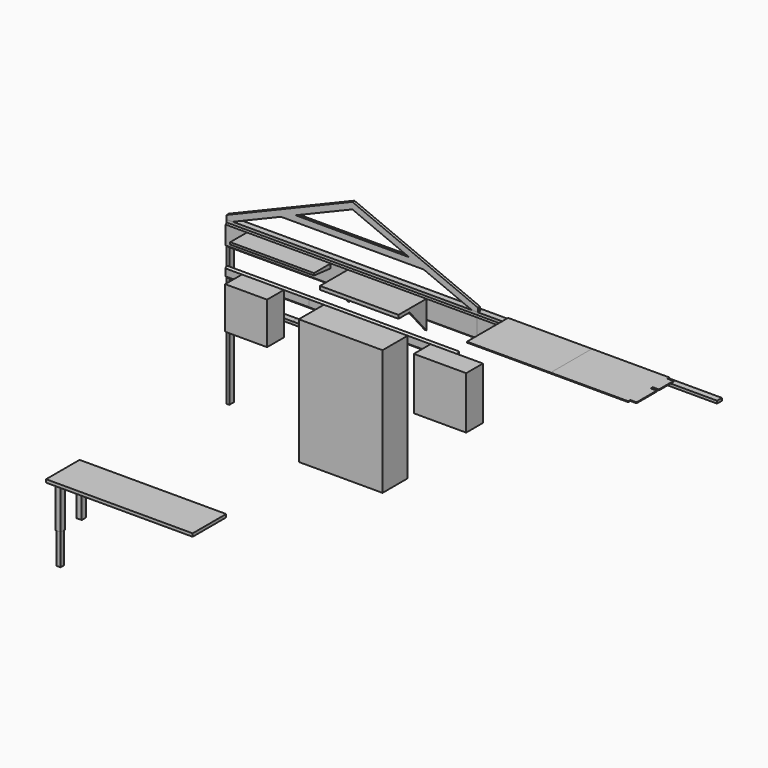
from build123d import *

# Parameters (mm, degrees)
F0_W      = 38.1
F0_H      = 88.9
F1_DEPTH  = 2324.1
F2_W      = 88.9
F2_H      = 38.1
F3_DEPTH  = 3657.6
F5_DEPTH  = 2438.4
F6_DEPTH  = 1219.2
F8_DEPTH  = 1219.2
F9_W      = 88.9
F9_H      = 38.1
F10_DEPTH = 914.4
F11_DEPTH = 1028.7
F12_DEPTH = 1028.7
F13_W     = 609.6
F13_H     = 609.6
F14_DEPTH = 304.8
F15_W     = 1219.2
F15_H     = 1828.8
F16_DEPTH = 457.2
F17_W     = 762
F17_H     = 762
F18_DEPTH = 304.8
F19_W     = 1219.2
F19_H     = 63.5
F20_DEPTH = 304.8
F22_DEPTH = 1529.2895152817
F23_W     = 1143
F23_H     = 50.8
F24_DEPTH = 508
F26_DEPTH = 25.4
F28_DEPTH = 25.4
F29_DEPTH = 1130.3
F30_W     = 1219.2
F30_H     = 749.3
F31_DEPTH = 12.7
F32_DEPTH = 3479.8
F33_DEPTH = 1130.3
F34_DEPTH = 635
F35_W     = 266.7
F35_H     = 12.7
F35_W_2   = 368.3
F36_DEPTH = 88.9
F37_W     = 2133.6
F37_H     = 609.6
F38_DEPTH = 44.45
F40_DEPTH = 38.1
F42_DEPTH = 6.35
F43_W     = 76.2
F43_H     = 76.2
F44_DEPTH = 609.6
F45_T     = -6.35
F46_W     = 58.42
F46_H     = 58.42
F47_DEPTH = 457.2
F48_T     = -2.54


with BuildPart() as f1:
    # F0 (on Top) → F1 (new body)
    with BuildSketch(Plane.XY):
        with Locations((19.05, -44.45)):
            Rectangle(F0_W, F0_H)
    extrude(amount=F1_DEPTH)


with BuildPart() as f3:
    # F2 (on face) → F3 (new body)
    with BuildSketch(Plane(origin=(0, 0, 0), x_dir=(0, -1, 0), z_dir=(-1, 0, 0))):
        with Locations((44.45, 2343.15)):
            Rectangle(F2_W, F2_H)
    extrude(amount=-F3_DEPTH)


with BuildPart() as f5:
    # F4 (on face) → F5 (new body)
    with BuildSketch(Plane(origin=(0, 0, 0), x_dir=(0, -1, 0), z_dir=(-1, 0, 0))):
        Polygon((107.95, 2305.05), (88.9, 2324.1), (88.9, 2019.3), (107.95, 2038.35), align=None)
    extrude(amount=-F5_DEPTH)


with BuildPart() as f6:
    # F6 (new): a face of the model
    f6_faces = [f5.part.faces().sort_by_distance(p)[0] for p in [
        (2438.4, -98.2133333333, 2171.7),
    ]]
    extrude(f6_faces, amount=F6_DEPTH)


with BuildPart() as f8:
    # F7 (on face) → F8 (new body)
    with BuildSketch(Plane(origin=(0, 0, 0), x_dir=(0, -1, 0), z_dir=(-1, 0, 0))):
        Polygon((114.3, 1747.0956106186), (88.9, 1772.4956106186), (88.9, 1620.0956106186), (114.3, 1645.4956106186), align=None)
    extrude(amount=-F8_DEPTH)


with BuildPart() as f10:
    # F9 (on face) → F10 (new body)
    with BuildSketch(Plane.YZ.offset(38.1)):
        with Locations((-44.45, 1349.1220453262)):
            Rectangle(F9_W, F9_H)
    extrude(amount=F10_DEPTH)


with BuildPart() as f11:
    # F11 (new): a face of the model
    f11_faces = [f6.part.faces().sort_by_distance(p)[0] for p in [
        (3657.6, -98.2133333333, 2171.7),
    ]]
    extrude(f11_faces, amount=F11_DEPTH)


with BuildPart() as f12:
    # F12 (new): a face of the model
    f12_faces = [f8.part.faces().sort_by_distance(p)[0] for p in [
        (1219.2, -100.7533333333, 1696.2956106186),
    ]]
    extrude(f12_faces, amount=F12_DEPTH)


with BuildPart() as f14:
    # F13 (on face) → F14 (new body)
    with BuildSketch(Plane.XZ.offset(114.3)):
        with Locations((546.8414686203, 1442.2956106186)):
            Rectangle(F13_W, F13_H)
    extrude(amount=F14_DEPTH)


with BuildPart() as f16:
    # F15 (on face) → F16 (new body)
    with BuildSketch(Plane.XZ.offset(114.3)):
        with Locations((2044.3823858261, 832.6956106186)):
            Rectangle(F15_W, F15_H)
    extrude(amount=F16_DEPTH)


with BuildPart() as f18:
    # F17 (on face) → F18 (new body)
    with BuildSketch(Plane.XZ.offset(114.3)):
        with Locations((3368.7196163048, 1366.0956106186)):
            Rectangle(F17_W, F17_H)
    extrude(amount=F18_DEPTH)


with BuildPart() as f20:
    # F19 (on face) → F20 (new body)
    with BuildSketch(Plane.XZ.offset(107.95)):
        with Locations((919.6885152817, 2273.3)):
            Rectangle(F19_W, F19_H)
    extrude(amount=F20_DEPTH)

    # F21 (on face) → F22 (cut, through all)
    with BuildSketch(Plane.YZ.offset(1529.2885152817)):
        Polygon((-107.95, 2241.55), (-412.75, 2273.3), (-412.75, 2241.55), align=None)
    extrude(amount=-F22_DEPTH, mode=Mode.SUBTRACT)


with BuildPart() as f24:
    # F23 (on face) → F24 (new body)
    with BuildSketch(Plane.XZ.offset(107.95)):
        with Locations((2350.8992757797, 2279.65)):
            Rectangle(F23_W, F23_H)
    extrude(amount=F24_DEPTH)

    # F25 (on face) → F26 (join)
    with BuildSketch(Plane.YZ.offset(2922.3992757797)):
        Polygon((-107.95, 1898.65), (-107.95, 2254.25), (-412.75, 2254.25), align=None)
    extrude(amount=-F26_DEPTH)

    # F27 (on face) → F28 (join)
    with BuildSketch(Plane(origin=(1779.3992757797, 0, 0), x_dir=(0, -1, 0), z_dir=(-1, 0, 0))):
        Polygon((107.95, 2254.25), (107.95, 1898.65), (412.75, 2254.25), align=None)
    extrude(amount=-F28_DEPTH)


with BuildPart() as f29:
    # F29 (new): a face of the model
    f29_faces = [f12.part.faces().sort_by_distance(p)[0] for p in [
        (2247.9, -100.7533333333, 1696.2956106186),
    ]]
    extrude(f29_faces, amount=F29_DEPTH)


with BuildPart() as f31:
    # F30 (on face) → F31 (new body)
    with BuildSketch(Plane.XY.offset(2362.2)):
        with Locations((4634.7321610946, -374.65)):
            Rectangle(F30_W, F30_H)
    extrude(amount=F31_DEPTH)


with BuildPart() as f32:
    # F32 (new): a face of the model
    f32_faces = [f3.part.faces().sort_by_distance(p)[0] for p in [
        (3657.6, -44.45, 2343.15),
    ]]
    extrude(f32_faces, amount=F32_DEPTH)


with BuildPart() as f33:
    # F33 (new): a face of the model
    f33_faces = [f31.part.faces().sort_by_distance(p)[0] for p in [
        (5244.3321610946, -374.65, 2368.55),
    ]]
    extrude(f33_faces, amount=F33_DEPTH)

    # F35 (on face) → F36 (join)
    with BuildSketch(Plane.YZ.offset(6374.6321610946)):
        with Locations((-171.45, 2368.55)):
            Rectangle(F35_W, F35_H)
        with Locations((-527.05, 2368.55)):
            Rectangle(F35_W_2, F35_H)
    extrude(amount=F36_DEPTH)


with BuildPart() as f34:
    # F34 (new): a face of the model
    f34_faces = [f10.part.faces().sort_by_distance(p)[0] for p in [
        (952.5, -44.45, 1349.1220453262),
    ]]
    extrude(f34_faces, amount=F34_DEPTH)


with BuildPart() as f38:
    # F37 (on Top) → F38 (new body)
    with BuildSketch(Plane.XY):
        with Locations((674.9990154266, -2581.2145842905)):
            Rectangle(F37_W, F37_H)
    extrude(amount=F38_DEPTH)


with BuildPart() as f40:
    # F39 (on face) → F40 (new body)
    with BuildSketch(Plane.XZ.offset(88.9)):
        Polygon((1828.8, 3183.4666666667), (0, 2421.4666666667), (0, 2362.2), (88.9, 2362.2), (789.94, 2654.3), (1003.3, 2743.2), (1828.8, 3087.1583333333), align=None)
        Polygon((3657.6, 2421.4666666667), (1828.8, 3183.4666666667), (1828.8, 3087.1583333333), (2654.3, 2743.2), (2867.66, 2654.3), (3263.9, 2489.2), (3568.7, 2362.2), (3657.6, 2362.2), align=None)
        Polygon((2654.3, 2743.2), (1828.8, 2743.2), (1828.8, 2654.3), (2867.66, 2654.3), align=None)
        Polygon((1828.8, 2654.3), (1828.8, 2743.2), (1003.3, 2743.2), (789.94, 2654.3), align=None)
    extrude(amount=-F40_DEPTH)


with BuildPart() as f42:
    # F41 (on face) → F42 (new body)
    with BuildSketch(Plane(origin=(0, 0, 0), x_dir=(1, 0, 0), z_dir=(0, 0, -1))):
        Polygon((-239.4009845734, 2809.8145842905), (-315.6009845734, 2809.8145842905), (-315.6009845734, 2581.2145842905), (-315.6009845734, 2352.6145842905), (-239.4009845734, 2352.6145842905), align=None)
    extrude(amount=F42_DEPTH)

    # F43 (on face) → F44 (join)
    with BuildSketch(Plane(origin=(0, 0, -6.35), x_dir=(1, 0, 0), z_dir=(0, 0, -1))):
        with Locations((-277.5009845734, 2771.7145842905)):
            Rectangle(F43_W, F43_H)
        with Locations((-277.5009845734, 2390.7145842905)):
            Rectangle(F43_W, F43_H)
    extrude(amount=F44_DEPTH)

    # F45
    f45_openings = [f42.faces().sort_by_distance(p)[0] for p in [
        (-277.500985, -2771.714584, -615.95),
        (-277.500985, -2390.714584, -615.95),
    ]]
    offset(amount=F45_T, openings=f45_openings, kind=Kind.INTERSECTION)


with BuildPart() as f47:
    # F46 (on face) → F47 (new body)
    with BuildSketch(Plane(origin=(0, 0, -615.95), x_dir=(1, 0, 0), z_dir=(0, 0, -1))):
        with Locations((-277.5009845734, 2771.7145842905)):
            Rectangle(F46_W, F46_H)
    extrude(amount=F47_DEPTH)

    # F48
    f48_openings = [f47.faces().sort_by_distance(p)[0] for p in [
        (-277.500985, -2771.714584, -615.95),
    ]]
    offset(amount=F48_T, openings=f48_openings)


solid = Compound([f1.part, f3.part, f5.part, f6.part, f8.part, f10.part, f11.part, f12.part, f14.part, f16.part, f18.part, f20.part, f24.part, f29.part, f31.part, f32.part, f33.part, f34.part, f38.part, f40.part, f42.part, f47.part])
